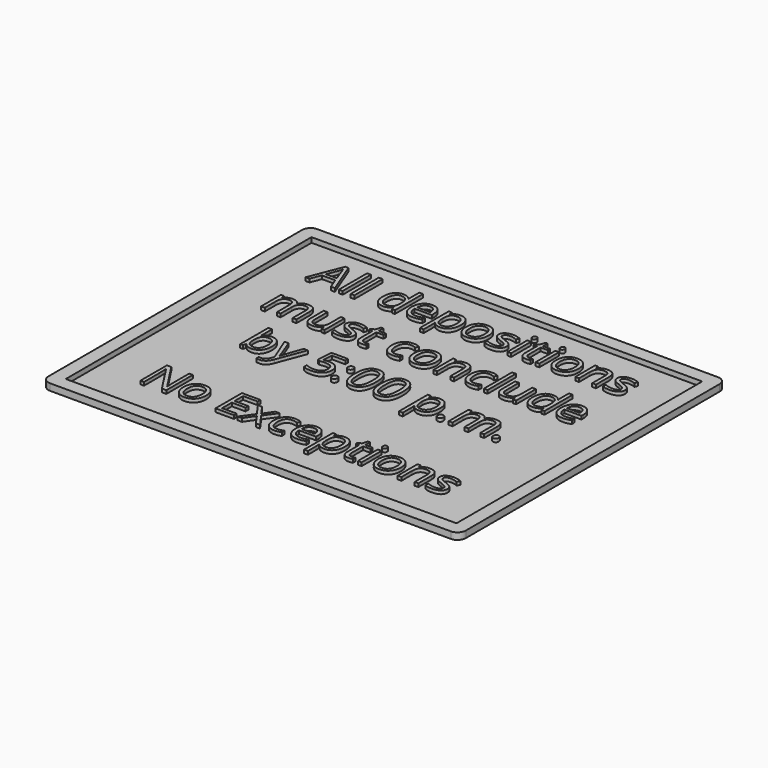
from build123d import *

# Parameters (mm, degrees)
F0_W         = 250
F0_H         = 200
F1_DEPTH     = 1
F2_TEXT_SIZE = 27.7777777778
F3_DEPTH     = 2
F4_W         = 250
F4_H         = 200
F4_W_2       = 234
F4_H_2       = 184
F5_DEPTH     = 3
F6_R         = 5


# Not quite as in the source:
# - Text() gives the source's letters only with a copy of the font that has no kerning and outlines rounded to 1/6400 em; it was checked with that copy


with BuildPart() as f1:
    # F0 (on Top) → F1 (new body)
    with BuildSketch(Plane.XY):
        with Locations((0, 25)):
            Rectangle(F0_W, F0_H)
    extrude(amount=F1_DEPTH)

    # F2 (on face) → F3 (join)
    with BuildSketch(Plane.XY.offset(1)):
        with Locations((-94.9869791667, 85)):
            Text('All depositions', F2_TEXT_SIZE, font='Open Sans', text_align=(TextAlign.LEFT, TextAlign.BOTTOM))
        with Locations((-95.234375, 49)):
            Text('must conclude', F2_TEXT_SIZE, font='Open Sans', text_align=(TextAlign.LEFT, TextAlign.BOTTOM))
        with Locations((-78.9366319444, 13)):
            Text('by 5:00 p.m.', F2_TEXT_SIZE, font='Open Sans', text_align=(TextAlign.LEFT, TextAlign.BOTTOM))
        with Locations((-92.6041666667, -45)):
            Text('No Exceptions', F2_TEXT_SIZE, font='Open Sans', text_align=(TextAlign.LEFT, TextAlign.BOTTOM))
    extrude(amount=F3_DEPTH)

    # F4 (on face) → F5 (join)
    with BuildSketch(Plane.XY.offset(1)):
        with Locations((0, 25)):
            Rectangle(F4_W, F4_H)
        with Locations((0, 25)):
            Rectangle(F4_W_2, F4_H_2, mode=Mode.SUBTRACT)
    extrude(amount=F5_DEPTH)

    # F6
    f6_edges = [f1.edges().sort_by_distance(p)[0] for p in [
        (-125, -75, 2),
        (-125, 125, 2),
        (125, 125, 2),
        (125, -75, 2),
    ]]
    fillet(f6_edges, radius=F6_R)


solid = f1.part
